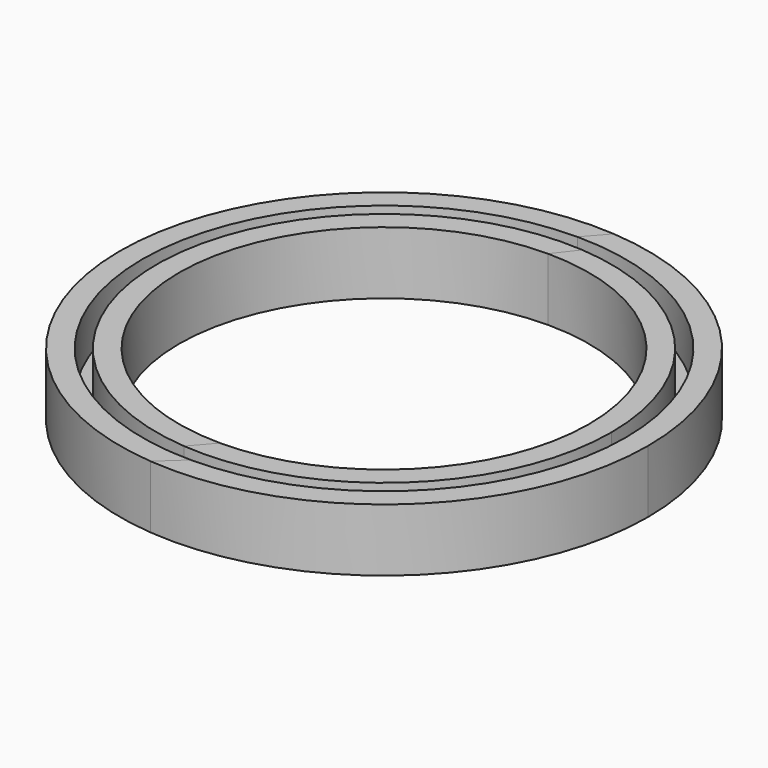
from build123d import *

# Parameters (mm, degrees)
F1_DEPTH = 7
F2_DEPTH = 7
F3_DEPTH = 2
F4_DEPTH = 2


with BuildPart() as f1:
    # F0 (on Top) → F1 (new body)
    with BuildSketch(Plane.XY):
        with BuildLine():
            ThreePointArc((-2.0932090565, -25.3136025853), (17.2045414058, -18.6859239808), (25.4, 0))
            ThreePointArc((25.4, 0), (18.6128618146, 17.2835579402), (1.8786318842, 25.33043115))
            Line((1.8786318842, 25.33043115), (0, 22.9))
            ThreePointArc((0, 22.9), (16.1927452892, 16.1927452892), (22.9, 0))
            ThreePointArc((22.9, 0), (16.1927452892, -16.1927452892), (0, -22.9))
            Line((0, -22.9), (-2.0932090565, -25.3136025853))
        make_face()
    extrude(amount=F1_DEPTH)



with BuildPart() as f1b:
    # F0 (on Top) → F1, piece 2 (new body)
    with BuildSketch(Plane.XY):
        with BuildLine():
            Line((2.1367751989, 29.4099787147), (0, 26.9875))
            ThreePointArc((0, 26.9875), (19.0830442573, 19.0830442573), (26.9875, 0))
            ThreePointArc((26.9875, 0), (19.0830442573, -19.0830442573), (0, -26.9875))
            Line((0, -26.9875), (-2.5972767503, -29.3728924305))
            ThreePointArc((-2.5972767503, -29.3728924305), (19.9113718522, -21.7497109685), (29.4875, 0))
            ThreePointArc((29.4875, 0), (21.5930638739, 20.0811416206), (2.1367751989, 29.4099787147))
        make_face()
    extrude(amount=F1_DEPTH)


with BuildPart() as f2:
    # F0 (on Top) → F2 (new body)
    with BuildSketch(Plane.XY):
        with BuildLine():
            ThreePointArc((0, -26.9875), (-26.9875, 0), (0, 26.9875))
            Line((0, 26.9875), (2.1367751989, 29.4099787147))
            ThreePointArc((2.1367751989, 29.4099787147), (-29.3923374443, 2.3670986064), (-2.5972767503, -29.3728924305))
            Line((-2.5972767503, -29.3728924305), (0, -26.9875))
        make_face()
    extrude(amount=F2_DEPTH)



with BuildPart() as f2b:
    # F0 (on Top) → F2, piece 2 (new body)
    with BuildSketch(Plane.XY):
        with BuildLine():
            Line((0, 22.9), (1.8786318842, 25.33043115))
            ThreePointArc((1.8786318842, 25.33043115), (-25.3222441558, 1.9859382958), (-2.0932090565, -25.3136025853))
            Line((-2.0932090565, -25.3136025853), (0, -22.9))
            ThreePointArc((0, -22.9), (-22.9, 0), (0, 22.9))
        make_face()
    extrude(amount=F2_DEPTH)


with BuildPart() as f1_1:
    add(f1.part)

    add(f1b.part)  # F3 merges F1b
    # F0 (on Top) → F3 (join)
    with BuildSketch(Plane.XY):
        with BuildLine():
            ThreePointArc((1.8786318842, 25.33043115), (18.6128618146, 17.2835579402), (25.4, 0))
            ThreePointArc((25.4, 0), (17.2045414058, -18.6859239808), (-2.0932090565, -25.3136025853))
            Line((-2.0932090565, -25.3136025853), (0, -26.9875))
            ThreePointArc((0, -26.9875), (19.0830442573, -19.0830442573), (26.9875, 0))
            ThreePointArc((26.9875, 0), (19.0830442573, 19.0830442573), (0, 26.9875))
            Line((0, 26.9875), (1.8786318842, 25.33043115))
        make_face()
    extrude(amount=F3_DEPTH)


with BuildPart() as f2_1:
    add(f2.part)

    add(f2b.part)  # F4 merges F2b
    # F0 (on Top) → F4 (join)
    with BuildSketch(Plane.XY):
        with BuildLine():
            ThreePointArc((-2.0932090565, -25.3136025853), (-25.3222441558, 1.9859382958), (1.8786318842, 25.33043115))
            Line((1.8786318842, 25.33043115), (0, 26.9875))
            ThreePointArc((0, 26.9875), (-26.9875, 0), (0, -26.9875))
            Line((0, -26.9875), (-2.0932090565, -25.3136025853))
        make_face()
    extrude(amount=F4_DEPTH)


solid = Compound([f1_1.part, f2_1.part])
